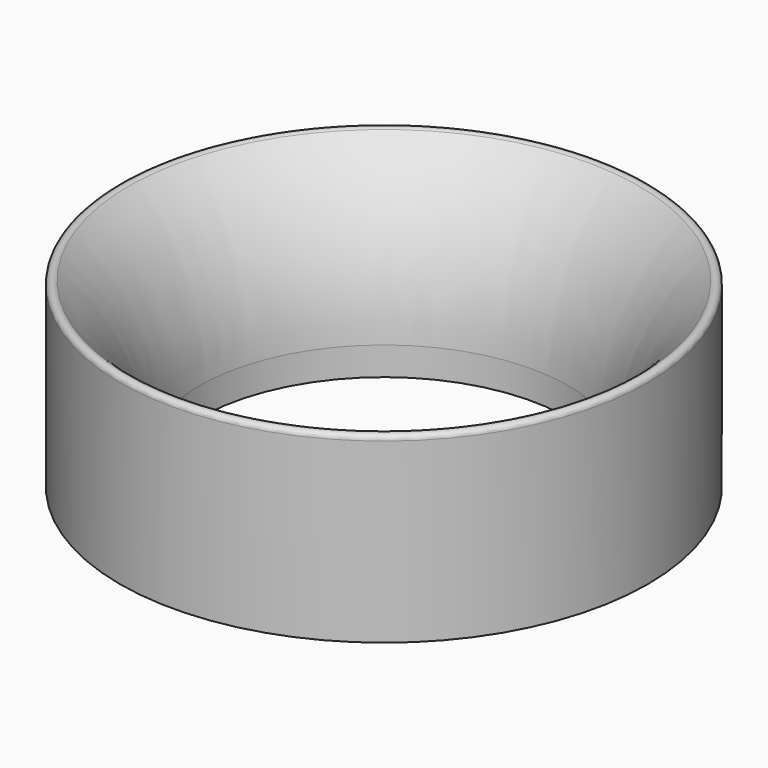
from build123d import *

# Parameters (mm, degrees)
F0_R     = 35
F0_R_2   = 24.5425
F1_DEPTH = 25
F3_R     = 0.7


# Not quite as in the source:
# - a fillet or chamfer that OpenCascade refuses, or shapes differently, is made with other operations: its cross-section is extruded or revolved along the edge and cut away or added


with BuildPart() as f1:
    # F0 (on Top) → F1 (new body)
    with BuildSketch(Plane.XY):
        Circle(F0_R)
        Circle(F0_R_2, mode=Mode.SUBTRACT)
    extrude(amount=F1_DEPTH)

    # F2: fillet of radius 26.7977705423 on 1 edges, made by hand

    # F2_s1 → F2_t2 (revolve, cut)
    with BuildSketch(Plane.XZ):
        with BuildLine():
            ThreePointArc((24.5425, 3.7605069589), (27.2986053896, 15.5976874814), (35, 25))
            Line((35, 25), (34.6731945892, 25.4247898608))
            ThreePointArc((34.6731945892, 25.4247898608), (29.77125, 25.5359554108), (24.5425, 25.5359554108))
            Line((24.5425, 25.5359554108), (24.0065445892, 25))
            Line((24.0065445892, 25), (24.0065445892, 3.7605069589))
            Line((24.0065445892, 3.7605069589), (24.5425, 3.7605069589))
        make_face()
    revolve(axis=Axis((0, 0, 25), (0, 0, 1)), mode=Mode.SUBTRACT)

    # F3
    f3_edges = [f1.edges().sort_by_distance(p)[0] for p in [
        (-35, 0, 25),
    ]]
    fillet(f3_edges, radius=F3_R)


solid = f1.part
